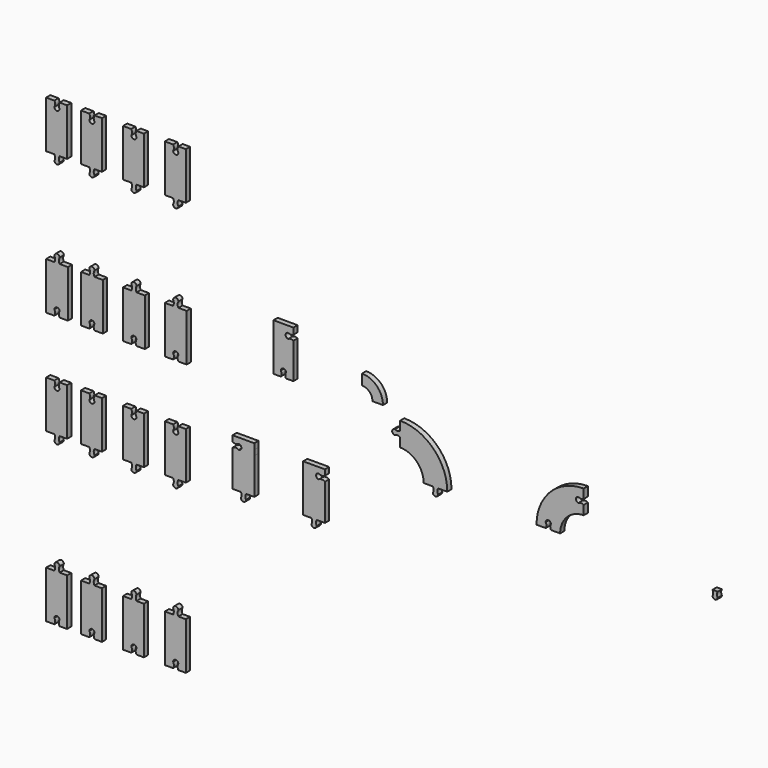
from build123d import *

# Parameters (mm, degrees)
F1_DEPTH = 25.4
F2_DEPTH = 25.4
F3_DEPTH = 25.4
F4_DEPTH = 25.4
F6_DEPTH = 25.4
F7_DEPTH = 25.4
F8_DEPTH = 25.4
F9_DEPTH = 25.4


# Not quite as in the source:
# - a feature names something its author has since deleted; it is built from what else it names


with BuildPart() as f1:
    # F0 (on Front) → F1 (new body)
    with BuildSketch(Plane.XZ):
        with BuildLine():
            Line((-45.9600600243, 819.565417695), (-82.0480443865, 819.565417695))
            ThreePointArc((-82.0480443865, 819.565417695), (-85.8930500594, 806.128817695), (-82.0480443865, 792.692217695))
            ThreePointArc((-82.0480443865, 792.692217695), (-94.7480443865, 779.992217695), (-107.4480443865, 792.692217695))
            ThreePointArc((-107.4480443865, 792.692217695), (-103.6030387136, 806.128817695), (-107.4480443865, 819.565417695))
            Line((-107.4480443865, 819.565417695), (-147.5600600243, 819.565417695))
            Line((-147.5600600243, 819.565417695), (-147.5600600243, 590.965417695))
            Line((-147.5600600243, 590.965417695), (-107.4480443865, 590.965417695))
            Line((-107.4480443865, 590.965417695), (-82.0480443865, 590.965417695))
            Line((-82.0480443865, 590.965417695), (-45.9600600243, 590.965417695))
            Line((-45.9600600243, 590.965417695), (-45.9600600243, 819.565417695))
        make_face()
    extrude(amount=F1_DEPTH)


with BuildPart() as f1b:
    # F0 (on Front) → F1, piece 2 (new body)
    with BuildSketch(Plane.XZ):
        with BuildLine():
            Line((21.4956142008, 590.965417695), (61.6076298386, 590.965417695))
            Line((61.6076298386, 590.965417695), (87.0076298386, 590.965417695))
            Line((87.0076298386, 590.965417695), (123.0956142008, 590.965417695))
            Line((123.0956142008, 590.965417695), (123.0956142008, 819.565417695))
            Line((123.0956142008, 819.565417695), (87.0076298386, 819.565417695))
            ThreePointArc((87.0076298386, 819.565417695), (83.1626241657, 806.128817695), (87.0076298386, 792.692217695))
            ThreePointArc((87.0076298386, 792.692217695), (74.3076298386, 779.992217695), (61.6076298386, 792.692217695))
            ThreePointArc((61.6076298386, 792.692217695), (65.4526355115, 806.128817695), (61.6076298386, 819.565417695))
            Line((61.6076298386, 819.565417695), (21.4956142008, 819.565417695))
            Line((21.4956142008, 819.565417695), (21.4956142008, 590.965417695))
        make_face()
    extrude(amount=F1_DEPTH)


with BuildPart() as f1c:
    # F0 (on Front) → F1, piece 3 (new body)
    with BuildSketch(Plane.XZ):
        with BuildLine():
            Line((264.7652149528, 590.965417695), (290.1652149528, 590.965417695))
            Line((290.1652149528, 590.965417695), (326.2531993151, 590.965417695))
            Line((326.2531993151, 590.965417695), (326.2531993151, 819.565417695))
            Line((326.2531993151, 819.565417695), (290.1652149528, 819.565417695))
            ThreePointArc((290.1652149528, 819.565417695), (286.3202092799, 806.128817695), (290.1652149528, 792.692217695))
            ThreePointArc((290.1652149528, 792.692217695), (277.4652149528, 779.992217695), (264.7652149528, 792.692217695))
            ThreePointArc((264.7652149528, 792.692217695), (268.6102206258, 806.128817695), (264.7652149528, 819.565417695))
            Line((264.7652149528, 819.565417695), (224.6531993151, 819.565417695))
            Line((224.6531993151, 819.565417695), (224.6531993151, 590.965417695))
            Line((224.6531993151, 590.965417695), (264.7652149528, 590.965417695))
        make_face()
    extrude(amount=F1_DEPTH)


with BuildPart() as f1d:
    # F0 (on Front) → F1, piece 4 (new body)
    with BuildSketch(Plane.XZ):
        with BuildLine():
            Line((427.3546077311, 590.965417695), (467.4666233689, 590.965417695))
            Line((467.4666233689, 590.965417695), (492.8666233689, 590.965417695))
            Line((492.8666233689, 590.965417695), (528.9546077311, 590.965417695))
            Line((528.9546077311, 590.965417695), (528.9546077311, 819.565417695))
            Line((528.9546077311, 819.565417695), (492.8666233689, 819.565417695))
            ThreePointArc((492.8666233689, 819.565417695), (489.0216176959, 806.128817695), (492.8666233689, 792.692217695))
            ThreePointArc((492.8666233689, 792.692217695), (480.1666233689, 779.992217695), (467.4666233689, 792.692217695))
            ThreePointArc((467.4666233689, 792.692217695), (471.3116290418, 806.128817695), (467.4666233689, 819.565417695))
            Line((467.4666233689, 819.565417695), (427.3546077311, 819.565417695))
            Line((427.3546077311, 819.565417695), (427.3546077311, 590.965417695))
        make_face()
    extrude(amount=F1_DEPTH)


with BuildPart() as f1e:
    # F0 (on Front) → F1, piece 5 (new body)
    with BuildSketch(Plane.XZ):
        with BuildLine():
            Line((492.8666233689, 131.5058790922), (467.4666233689, 131.5058790922))
            Line((467.4666233689, 131.5058790922), (427.3546077311, 131.5058790922))
            Line((427.3546077311, 131.5058790922), (427.3546077311, -97.0941209078))
            Line((427.3546077311, -97.0941209078), (467.4666233689, -97.0941209078))
            ThreePointArc((467.4666233689, -97.0941209078), (471.3116290418, -83.6575209078), (467.4666233689, -70.2209209078))
            ThreePointArc((467.4666233689, -70.2209209078), (480.1666233689, -57.5209209078), (492.8666233689, -70.2209209078))
            ThreePointArc((492.8666233689, -70.2209209078), (489.0216176959, -83.6575209078), (492.8666233689, -97.0941209078))
            Line((492.8666233689, -97.0941209078), (532.9786390066, -97.0941209078))
            Line((532.9786390066, -97.0941209078), (532.9786390066, 131.5058790922))
            Line((532.9786390066, 131.5058790922), (492.8666233689, 131.5058790922))
        make_face()
    extrude(amount=F1_DEPTH)


with BuildPart() as f1f:
    # F0 (on Front) → F1, piece 6 (new body)
    with BuildSketch(Plane.XZ):
        with BuildLine():
            ThreePointArc((264.7652149528, -70.2209209078), (277.4652149528, -57.5209209078), (290.1652149528, -70.2209209078))
            ThreePointArc((290.1652149528, -70.2209209078), (286.3202092799, -83.6575209078), (290.1652149528, -97.0941209078))
            Line((290.1652149528, -97.0941209078), (330.2772305906, -97.0941209078))
            Line((330.2772305906, -97.0941209078), (330.2772305906, 131.5058790922))
            Line((330.2772305906, 131.5058790922), (290.1652149528, 131.5058790922))
            Line((290.1652149528, 131.5058790922), (264.7652149528, 131.5058790922))
            Line((264.7652149528, 131.5058790922), (224.6531993151, 131.5058790922))
            Line((224.6531993151, 131.5058790922), (224.6531993151, -97.0941209078))
            Line((224.6531993151, -97.0941209078), (264.7652149528, -97.0941209078))
            ThreePointArc((264.7652149528, -97.0941209078), (268.6102206258, -83.6575209078), (264.7652149528, -70.2209209078))
        make_face()
    extrude(amount=F1_DEPTH)


with BuildPart() as f1g:
    # F0 (on Front) → F1, piece 7 (new body)
    with BuildSketch(Plane.XZ):
        with BuildLine():
            Line((21.4956142008, -97.0941209078), (61.6076298386, -97.0941209078))
            ThreePointArc((61.6076298386, -97.0941209078), (65.4526355115, -83.6575209078), (61.6076298386, -70.2209209078))
            ThreePointArc((61.6076298386, -70.2209209078), (74.3076298386, -57.5209209078), (87.0076298386, -70.2209209078))
            ThreePointArc((87.0076298386, -70.2209209078), (83.1626241657, -83.6575209078), (87.0076298386, -97.0941209078))
            Line((87.0076298386, -97.0941209078), (127.1196454763, -97.0941209078))
            Line((127.1196454763, -97.0941209078), (127.1196454763, 131.5058790922))
            Line((127.1196454763, 131.5058790922), (87.0076298386, 131.5058790922))
            Line((87.0076298386, 131.5058790922), (61.6076298386, 131.5058790922))
            Line((61.6076298386, 131.5058790922), (21.4956142008, 131.5058790922))
            Line((21.4956142008, 131.5058790922), (21.4956142008, -97.0941209078))
        make_face()
    extrude(amount=F1_DEPTH)


with BuildPart() as f1h:
    # F0 (on Front) → F1, piece 8 (new body)
    with BuildSketch(Plane.XZ):
        with BuildLine():
            Line((-107.4480443865, 131.5058790922), (-147.5600600243, 131.5058790922))
            Line((-147.5600600243, 131.5058790922), (-147.5600600243, -97.0941209078))
            Line((-147.5600600243, -97.0941209078), (-107.4480443865, -97.0941209078))
            ThreePointArc((-107.4480443865, -97.0941209078), (-103.6030387136, -83.6575209078), (-107.4480443865, -70.2209209078))
            ThreePointArc((-107.4480443865, -70.2209209078), (-94.7480443865, -57.5209209078), (-82.0480443865, -70.2209209078))
            ThreePointArc((-82.0480443865, -70.2209209078), (-85.8930500594, -83.6575209078), (-82.0480443865, -97.0941209078))
            Line((-82.0480443865, -97.0941209078), (-41.9360287488, -97.0941209078))
            Line((-41.9360287488, -97.0941209078), (-41.9360287488, 131.5058790922))
            Line((-41.9360287488, 131.5058790922), (-82.0480443865, 131.5058790922))
            Line((-82.0480443865, 131.5058790922), (-107.4480443865, 131.5058790922))
        make_face()
    extrude(amount=F1_DEPTH)


with BuildPart() as f1i:
    # F0 (on Front) → F1, piece 9 (new body)
    with BuildSketch(Plane.XZ):
        with BuildLine():
            ThreePointArc((-107.4480443865, -400.1181687243), (-103.6030387136, -386.6815687243), (-107.4480443865, -373.2449687243))
            Line((-107.4480443865, -373.2449687243), (-147.5600600243, -373.2449687243))
            Line((-147.5600600243, -373.2449687243), (-147.5600600243, -601.8449687243))
            Line((-147.5600600243, -601.8449687243), (-107.4480443865, -601.8449687243))
            Line((-107.4480443865, -601.8449687243), (-82.0480443865, -601.8449687243))
            Line((-82.0480443865, -601.8449687243), (-45.9600600243, -601.8449687243))
            Line((-45.9600600243, -601.8449687243), (-45.9600600243, -373.2449687243))
            Line((-45.9600600243, -373.2449687243), (-82.0480443865, -373.2449687243))
            ThreePointArc((-82.0480443865, -373.2449687243), (-85.8930500594, -386.6815687243), (-82.0480443865, -400.1181687243))
            ThreePointArc((-82.0480443865, -400.1181687243), (-94.7480443865, -412.8181687243), (-107.4480443865, -400.1181687243))
        make_face()
    extrude(amount=F1_DEPTH)


with BuildPart() as f1j:
    # F0 (on Front) → F1, piece 10 (new body)
    with BuildSketch(Plane.XZ):
        with BuildLine():
            ThreePointArc((61.6076298386, -400.1181687243), (65.4526355115, -386.6815687243), (61.6076298386, -373.2449687243))
            Line((61.6076298386, -373.2449687243), (21.4956142008, -373.2449687243))
            Line((21.4956142008, -373.2449687243), (21.4956142008, -601.8449687243))
            Line((21.4956142008, -601.8449687243), (61.6076298386, -601.8449687243))
            Line((61.6076298386, -601.8449687243), (87.0076298386, -601.8449687243))
            Line((87.0076298386, -601.8449687243), (123.0956142008, -601.8449687243))
            Line((123.0956142008, -601.8449687243), (123.0956142008, -373.2449687243))
            Line((123.0956142008, -373.2449687243), (87.0076298386, -373.2449687243))
            ThreePointArc((87.0076298386, -373.2449687243), (83.1626241657, -386.6815687243), (87.0076298386, -400.1181687243))
            ThreePointArc((87.0076298386, -400.1181687243), (74.3076298386, -412.8181687243), (61.6076298386, -400.1181687243))
        make_face()
    extrude(amount=F1_DEPTH)


with BuildPart() as f1k:
    # F0 (on Front) → F1, piece 11 (new body)
    with BuildSketch(Plane.XZ):
        with BuildLine():
            ThreePointArc((264.7652149528, -400.1181687243), (268.6102206258, -386.6815687243), (264.7652149528, -373.2449687243))
            Line((264.7652149528, -373.2449687243), (224.6531993151, -373.2449687243))
            Line((224.6531993151, -373.2449687243), (224.6531993151, -601.8449687243))
            Line((224.6531993151, -601.8449687243), (264.7652149528, -601.8449687243))
            Line((264.7652149528, -601.8449687243), (290.1652149528, -601.8449687243))
            Line((290.1652149528, -601.8449687243), (326.2531993151, -601.8449687243))
            Line((326.2531993151, -601.8449687243), (326.2531993151, -373.2449687243))
            Line((326.2531993151, -373.2449687243), (290.1652149528, -373.2449687243))
            ThreePointArc((290.1652149528, -373.2449687243), (286.3202092799, -386.6815687243), (290.1652149528, -400.1181687243))
            ThreePointArc((290.1652149528, -400.1181687243), (277.4652149528, -412.8181687243), (264.7652149528, -400.1181687243))
        make_face()
    extrude(amount=F1_DEPTH)


with BuildPart() as f1l:
    # F0 (on Front) → F1, piece 12 (new body)
    with BuildSketch(Plane.XZ):
        with BuildLine():
            Line((528.9546077311, -373.2449687243), (492.8666233689, -373.2449687243))
            ThreePointArc((492.8666233689, -373.2449687243), (489.0216176959, -386.6815687243), (492.8666233689, -400.1181687243))
            ThreePointArc((492.8666233689, -400.1181687243), (480.1666233689, -412.8181687243), (467.4666233689, -400.1181687243))
            ThreePointArc((467.4666233689, -400.1181687243), (471.3116290418, -386.6815687243), (467.4666233689, -373.2449687243))
            Line((467.4666233689, -373.2449687243), (427.3546077311, -373.2449687243))
            Line((427.3546077311, -373.2449687243), (427.3546077311, -601.8449687243))
            Line((427.3546077311, -601.8449687243), (467.4666233689, -601.8449687243))
            Line((467.4666233689, -601.8449687243), (492.8666233689, -601.8449687243))
            Line((492.8666233689, -601.8449687243), (528.9546077311, -601.8449687243))
            Line((528.9546077311, -601.8449687243), (528.9546077311, -373.2449687243))
        make_face()
    extrude(amount=F1_DEPTH)


with BuildPart() as f1m:
    # F0 (on Front) → F1, piece 13 (new body)
    with BuildSketch(Plane.XZ):
        with BuildLine():
            ThreePointArc((492.8666233689, -1385.466757881), (489.0216176959, -1398.903357881), (492.8666233689, -1412.339957881))
            Line((492.8666233689, -1412.339957881), (528.9546077311, -1412.339957881))
            Line((528.9546077311, -1412.339957881), (528.9546077311, -1183.739957881))
            Line((528.9546077311, -1183.739957881), (492.8666233689, -1183.739957881))
            Line((492.8666233689, -1183.739957881), (467.4666233689, -1183.739957881))
            Line((467.4666233689, -1183.739957881), (427.3546077311, -1183.739957881))
            Line((427.3546077311, -1183.739957881), (427.3546077311, -1412.339957881))
            Line((427.3546077311, -1412.339957881), (467.4666233689, -1412.339957881))
            ThreePointArc((467.4666233689, -1412.339957881), (471.3116290418, -1398.903357881), (467.4666233689, -1385.466757881))
            ThreePointArc((467.4666233689, -1385.466757881), (480.1666233689, -1372.766757881), (492.8666233689, -1385.466757881))
        make_face()
    extrude(amount=F1_DEPTH)


with BuildPart() as f1n:
    # F0 (on Front) → F1, piece 14 (new body)
    with BuildSketch(Plane.XZ):
        with BuildLine():
            ThreePointArc((264.7652149528, -1385.466757881), (277.4652149528, -1372.766757881), (290.1652149528, -1385.466757881))
            ThreePointArc((290.1652149528, -1385.466757881), (286.3202092799, -1398.903357881), (290.1652149528, -1412.339957881))
            Line((290.1652149528, -1412.339957881), (326.2531993151, -1412.339957881))
            Line((326.2531993151, -1412.339957881), (326.2531993151, -1183.739957881))
            Line((326.2531993151, -1183.739957881), (290.1652149528, -1183.739957881))
            Line((290.1652149528, -1183.739957881), (264.7652149528, -1183.739957881))
            Line((264.7652149528, -1183.739957881), (224.6531993151, -1183.739957881))
            Line((224.6531993151, -1183.739957881), (224.6531993151, -1412.339957881))
            Line((224.6531993151, -1412.339957881), (264.7652149528, -1412.339957881))
            ThreePointArc((264.7652149528, -1412.339957881), (268.6102206258, -1398.903357881), (264.7652149528, -1385.466757881))
        make_face()
    extrude(amount=F1_DEPTH)


with BuildPart() as f1o:
    # F0 (on Front) → F1, piece 15 (new body)
    with BuildSketch(Plane.XZ):
        with BuildLine():
            Line((87.0076298386, -1183.739957881), (61.6076298386, -1183.739957881))
            Line((61.6076298386, -1183.739957881), (21.4956142008, -1183.739957881))
            Line((21.4956142008, -1183.739957881), (21.4956142008, -1412.339957881))
            Line((21.4956142008, -1412.339957881), (61.6076298386, -1412.339957881))
            ThreePointArc((61.6076298386, -1412.339957881), (65.4526355115, -1398.903357881), (61.6076298386, -1385.466757881))
            ThreePointArc((61.6076298386, -1385.466757881), (74.3076298386, -1372.766757881), (87.0076298386, -1385.466757881))
            ThreePointArc((87.0076298386, -1385.466757881), (83.1626241657, -1398.903357881), (87.0076298386, -1412.339957881))
            Line((87.0076298386, -1412.339957881), (123.0956142008, -1412.339957881))
            Line((123.0956142008, -1412.339957881), (123.0956142008, -1183.739957881))
            Line((123.0956142008, -1183.739957881), (87.0076298386, -1183.739957881))
        make_face()
    extrude(amount=F1_DEPTH)


with BuildPart() as f1p:
    # F0 (on Front) → F1, piece 16 (new body)
    with BuildSketch(Plane.XZ):
        with BuildLine():
            ThreePointArc((-107.4480443865, -1385.466757881), (-94.7480443865, -1372.766757881), (-82.0480443865, -1385.466757881))
            ThreePointArc((-82.0480443865, -1385.466757881), (-85.8930500594, -1398.903357881), (-82.0480443865, -1412.339957881))
            Line((-82.0480443865, -1412.339957881), (-45.9600600243, -1412.339957881))
            Line((-45.9600600243, -1412.339957881), (-45.9600600243, -1183.739957881))
            Line((-45.9600600243, -1183.739957881), (-82.0480443865, -1183.739957881))
            Line((-82.0480443865, -1183.739957881), (-107.4480443865, -1183.739957881))
            Line((-107.4480443865, -1183.739957881), (-147.5600600243, -1183.739957881))
            Line((-147.5600600243, -1183.739957881), (-147.5600600243, -1412.339957881))
            Line((-147.5600600243, -1412.339957881), (-107.4480443865, -1412.339957881))
            ThreePointArc((-107.4480443865, -1412.339957881), (-103.6030387136, -1398.903357881), (-107.4480443865, -1385.466757881))
        make_face()
    extrude(amount=F1_DEPTH)


with BuildPart() as f2:
    # F0 (on Front) → F2 (new body)
    with BuildSketch(Plane.XZ):
        with BuildLine():
            ThreePointArc((492.8666233689, 158.3865135908), (480.1666233689, 171.0865135908), (467.4666233689, 158.3865135908))
            ThreePointArc((467.4666233689, 158.3865135908), (470.8542959546, 144.9461963415), (467.4666233689, 131.5058790922))
            Line((467.4666233689, 131.5058790922), (492.8666233689, 131.5058790922))
            ThreePointArc((492.8666233689, 131.5058790922), (489.0193000527, 144.9461963415), (492.8666233689, 158.3865135908))
        make_face()
    extrude(amount=F2_DEPTH)


with BuildPart() as f2b:
    # F0 (on Front) → F2, piece 2 (new body)
    with BuildSketch(Plane.XZ):
        with BuildLine():
            Line((264.7652149528, 131.5058790922), (290.1652149528, 131.5058790922))
            ThreePointArc((290.1652149528, 131.5058790922), (286.7775423671, 144.9461963415), (290.1652149528, 158.3865135908))
            ThreePointArc((290.1652149528, 158.3865135908), (277.4652149528, 171.0865135908), (264.7652149528, 158.3865135908))
            ThreePointArc((264.7652149528, 158.3865135908), (268.612538269, 144.9461963415), (264.7652149528, 131.5058790922))
        make_face()
    extrude(amount=F2_DEPTH)


with BuildPart() as f2c:
    # F0 (on Front) → F2, piece 3 (new body)
    with BuildSketch(Plane.XZ):
        with BuildLine():
            ThreePointArc((61.6076298386, 158.3865135908), (64.9953024243, 144.9461963415), (61.6076298386, 131.5058790922))
            Line((61.6076298386, 131.5058790922), (87.0076298386, 131.5058790922))
            ThreePointArc((87.0076298386, 131.5058790922), (83.1603065224, 144.9461963415), (87.0076298386, 158.3865135908))
            ThreePointArc((87.0076298386, 158.3865135908), (74.3076298386, 171.0865135908), (61.6076298386, 158.3865135908))
        make_face()
    extrude(amount=F2_DEPTH)


with BuildPart() as f2d:
    # F0 (on Front) → F2, piece 4 (new body)
    with BuildSketch(Plane.XZ):
        with BuildLine():
            ThreePointArc((-107.4480443865, 158.3865135908), (-103.6007210703, 144.9461963415), (-107.4480443865, 131.5058790922))
            Line((-107.4480443865, 131.5058790922), (-82.0480443865, 131.5058790922))
            ThreePointArc((-82.0480443865, 131.5058790922), (-85.4357169722, 144.9461963415), (-82.0480443865, 158.3865135908))
            ThreePointArc((-82.0480443865, 158.3865135908), (-94.7480443865, 171.0865135908), (-107.4480443865, 158.3865135908))
        make_face()
    extrude(amount=F2_DEPTH)


with BuildPart() as f2e:
    # F0 (on Front) → F2, piece 5 (new body)
    with BuildSketch(Plane.XZ):
        with BuildLine():
            Line((-82.0480443865, -601.8449687243), (-107.4480443865, -601.8449687243))
            ThreePointArc((-107.4480443865, -601.8449687243), (-103.6007210703, -615.2852859735), (-107.4480443865, -628.7256032228))
            ThreePointArc((-107.4480443865, -628.7256032228), (-94.7480443865, -641.4256032228), (-82.0480443865, -628.7256032228))
            ThreePointArc((-82.0480443865, -628.7256032228), (-85.4357169722, -615.2852859735), (-82.0480443865, -601.8449687243))
        make_face()
    extrude(amount=F2_DEPTH)


with BuildPart() as f2f:
    # F0 (on Front) → F2, piece 6 (new body)
    with BuildSketch(Plane.XZ):
        with BuildLine():
            Line((87.0076298386, -601.8449687243), (61.6076298386, -601.8449687243))
            ThreePointArc((61.6076298386, -601.8449687243), (64.9953024243, -615.2852859735), (61.6076298386, -628.7256032228))
            ThreePointArc((61.6076298386, -628.7256032228), (74.3076298386, -641.4256032228), (87.0076298386, -628.7256032228))
            ThreePointArc((87.0076298386, -628.7256032228), (83.1603065224, -615.2852859735), (87.0076298386, -601.8449687243))
        make_face()
    extrude(amount=F2_DEPTH)


with BuildPart() as f2g:
    # F0 (on Front) → F2, piece 7 (new body)
    with BuildSketch(Plane.XZ):
        with BuildLine():
            Line((290.1652149528, -601.8449687243), (264.7652149528, -601.8449687243))
            ThreePointArc((264.7652149528, -601.8449687243), (268.612538269, -615.2852859735), (264.7652149528, -628.7256032228))
            ThreePointArc((264.7652149528, -628.7256032228), (277.4652149528, -641.4256032228), (290.1652149528, -628.7256032228))
            ThreePointArc((290.1652149528, -628.7256032228), (286.7775423671, -615.2852859735), (290.1652149528, -601.8449687243))
        make_face()
    extrude(amount=F2_DEPTH)


with BuildPart() as f2h:
    # F0 (on Front) → F2, piece 8 (new body)
    with BuildSketch(Plane.XZ):
        with BuildLine():
            ThreePointArc((492.8666233689, -628.7256032228), (489.0193000527, -615.2852859735), (492.8666233689, -601.8449687243))
            Line((492.8666233689, -601.8449687243), (467.4666233689, -601.8449687243))
            ThreePointArc((467.4666233689, -601.8449687243), (470.8542959546, -615.2852859735), (467.4666233689, -628.7256032228))
            ThreePointArc((467.4666233689, -628.7256032228), (480.1666233689, -641.4256032228), (492.8666233689, -628.7256032228))
        make_face()
    extrude(amount=F2_DEPTH)


with BuildPart() as f2i:
    # F0 (on Front) → F2, piece 9 (new body)
    with BuildSketch(Plane.XZ):
        with BuildLine():
            Line((467.4666233689, -1183.739957881), (492.8666233689, -1183.739957881))
            ThreePointArc((492.8666233689, -1183.739957881), (489.0193000527, -1170.2996406317), (492.8666233689, -1156.8593233824))
            ThreePointArc((492.8666233689, -1156.8593233824), (480.1666233689, -1144.1593233824), (467.4666233689, -1156.8593233824))
            ThreePointArc((467.4666233689, -1156.8593233824), (470.8542959546, -1170.2996406317), (467.4666233689, -1183.739957881))
        make_face()
    extrude(amount=F2_DEPTH)


with BuildPart() as f2j:
    # F0 (on Front) → F2, piece 10 (new body)
    with BuildSketch(Plane.XZ):
        with BuildLine():
            Line((264.7652149528, -1183.739957881), (290.1652149528, -1183.739957881))
            ThreePointArc((290.1652149528, -1183.739957881), (286.7775423671, -1170.2996406317), (290.1652149528, -1156.8593233824))
            ThreePointArc((290.1652149528, -1156.8593233824), (277.4652149528, -1144.1593233824), (264.7652149528, -1156.8593233824))
            ThreePointArc((264.7652149528, -1156.8593233824), (268.612538269, -1170.2996406317), (264.7652149528, -1183.739957881))
        make_face()
    extrude(amount=F2_DEPTH)


with BuildPart() as f2k:
    # F0 (on Front) → F2, piece 11 (new body)
    with BuildSketch(Plane.XZ):
        with BuildLine():
            ThreePointArc((87.0076298386, -1156.8593233824), (74.3076298386, -1144.1593233824), (61.6076298386, -1156.8593233824))
            ThreePointArc((61.6076298386, -1156.8593233824), (64.9953024243, -1170.2996406317), (61.6076298386, -1183.739957881))
            Line((61.6076298386, -1183.739957881), (87.0076298386, -1183.739957881))
            ThreePointArc((87.0076298386, -1183.739957881), (83.1603065224, -1170.2996406317), (87.0076298386, -1156.8593233824))
        make_face()
    extrude(amount=F2_DEPTH)


with BuildPart() as f2l:
    # F0 (on Front) → F2, piece 12 (new body)
    with BuildSketch(Plane.XZ):
        with BuildLine():
            Line((-107.4480443865, -1183.739957881), (-82.0480443865, -1183.739957881))
            ThreePointArc((-82.0480443865, -1183.739957881), (-85.4357169722, -1170.2996406317), (-82.0480443865, -1156.8593233824))
            ThreePointArc((-82.0480443865, -1156.8593233824), (-94.7480443865, -1144.1593233824), (-107.4480443865, -1156.8593233824))
            ThreePointArc((-107.4480443865, -1156.8593233824), (-103.6007210703, -1170.2996406317), (-107.4480443865, -1183.739957881))
        make_face()
    extrude(amount=F2_DEPTH)


with BuildPart() as f2m:
    # F0 (on Front) → F2, piece 13 (new body)
    with BuildSketch(Plane.XZ):
        with BuildLine():
            ThreePointArc((467.4666233689, 590.965417695), (470.8542959546, 577.5251004457), (467.4666233689, 564.0847831964))
            ThreePointArc((467.4666233689, 564.0847831964), (480.1666233689, 551.3847831964), (492.8666233689, 564.0847831964))
            ThreePointArc((492.8666233689, 564.0847831964), (489.0193000527, 577.5251004457), (492.8666233689, 590.965417695))
            Line((492.8666233689, 590.965417695), (467.4666233689, 590.965417695))
        make_face()
    extrude(amount=F2_DEPTH)


with BuildPart() as f2n:
    # F0 (on Front) → F2, piece 14 (new body)
    with BuildSketch(Plane.XZ):
        with BuildLine():
            ThreePointArc((264.7652149528, 564.0847831964), (277.4652149528, 551.3847831964), (290.1652149528, 564.0847831964))
            ThreePointArc((290.1652149528, 564.0847831964), (286.7775423671, 577.5251004457), (290.1652149528, 590.965417695))
            Line((290.1652149528, 590.965417695), (264.7652149528, 590.965417695))
            ThreePointArc((264.7652149528, 590.965417695), (268.612538269, 577.5251004457), (264.7652149528, 564.0847831964))
        make_face()
    extrude(amount=F2_DEPTH)


with BuildPart() as f2o:
    # F0 (on Front) → F2, piece 15 (new body)
    with BuildSketch(Plane.XZ):
        with BuildLine():
            ThreePointArc((61.6076298386, 590.965417695), (64.9953024243, 577.5251004457), (61.6076298386, 564.0847831964))
            ThreePointArc((61.6076298386, 564.0847831964), (74.3076298386, 551.3847831964), (87.0076298386, 564.0847831964))
            ThreePointArc((87.0076298386, 564.0847831964), (83.1603065224, 577.5251004457), (87.0076298386, 590.965417695))
            Line((87.0076298386, 590.965417695), (61.6076298386, 590.965417695))
        make_face()
    extrude(amount=F2_DEPTH)


with BuildPart() as f2p:
    # F0 (on Front) → F2, piece 16 (new body)
    with BuildSketch(Plane.XZ):
        with BuildLine():
            ThreePointArc((-82.0480443865, 564.0847831964), (-85.4357169722, 577.5251004457), (-82.0480443865, 590.965417695))
            Line((-82.0480443865, 590.965417695), (-107.4480443865, 590.965417695))
            ThreePointArc((-107.4480443865, 590.965417695), (-103.6007210703, 577.5251004457), (-107.4480443865, 564.0847831964))
            ThreePointArc((-107.4480443865, 564.0847831964), (-94.7480443865, 551.3847831964), (-82.0480443865, 564.0847831964))
        make_face()
    extrude(amount=F2_DEPTH)


with BuildPart() as f3:
    # F0 (on Front) → F3 (new body)
    with BuildSketch(Plane.XZ):
        with BuildLine():
            Line((-107.4480443865, 131.5058790922), (-147.5600600243, 131.5058790922))
            Line((-147.5600600243, 131.5058790922), (-147.5600600243, -97.0941209078))
            Line((-147.5600600243, -97.0941209078), (-107.4480443865, -97.0941209078))
            ThreePointArc((-107.4480443865, -97.0941209078), (-103.6030387136, -83.6575209078), (-107.4480443865, -70.2209209078))
            ThreePointArc((-107.4480443865, -70.2209209078), (-94.7480443865, -57.5209209078), (-82.0480443865, -70.2209209078))
            ThreePointArc((-82.0480443865, -70.2209209078), (-85.8930500594, -83.6575209078), (-82.0480443865, -97.0941209078))
            Line((-82.0480443865, -97.0941209078), (-41.9360287488, -97.0941209078))
            Line((-41.9360287488, -97.0941209078), (-41.9360287488, 131.5058790922))
            Line((-41.9360287488, 131.5058790922), (-82.0480443865, 131.5058790922))
            Line((-82.0480443865, 131.5058790922), (-107.4480443865, 131.5058790922))
        make_face()
        with BuildLine():
            ThreePointArc((-107.4480443865, 158.3865135908), (-103.6007210703, 144.9461963415), (-107.4480443865, 131.5058790922))
            Line((-107.4480443865, 131.5058790922), (-82.0480443865, 131.5058790922))
            ThreePointArc((-82.0480443865, 131.5058790922), (-85.4357169722, 144.9461963415), (-82.0480443865, 158.3865135908))
            ThreePointArc((-82.0480443865, 158.3865135908), (-94.7480443865, 171.0865135908), (-107.4480443865, 158.3865135908))
        make_face()
    extrude(amount=F3_DEPTH)


with BuildPart() as f3b:
    # F0 (on Front) → F3, piece 2 (new body)
    with BuildSketch(Plane.XZ):
        with BuildLine():
            Line((21.4956142008, -97.0941209078), (61.6076298386, -97.0941209078))
            ThreePointArc((61.6076298386, -97.0941209078), (65.4526355115, -83.6575209078), (61.6076298386, -70.2209209078))
            ThreePointArc((61.6076298386, -70.2209209078), (74.3076298386, -57.5209209078), (87.0076298386, -70.2209209078))
            ThreePointArc((87.0076298386, -70.2209209078), (83.1626241657, -83.6575209078), (87.0076298386, -97.0941209078))
            Line((87.0076298386, -97.0941209078), (127.1196454763, -97.0941209078))
            Line((127.1196454763, -97.0941209078), (127.1196454763, 131.5058790922))
            Line((127.1196454763, 131.5058790922), (87.0076298386, 131.5058790922))
            Line((87.0076298386, 131.5058790922), (61.6076298386, 131.5058790922))
            Line((61.6076298386, 131.5058790922), (21.4956142008, 131.5058790922))
            Line((21.4956142008, 131.5058790922), (21.4956142008, -97.0941209078))
        make_face()
        with BuildLine():
            ThreePointArc((61.6076298386, 158.3865135908), (64.9953024243, 144.9461963415), (61.6076298386, 131.5058790922))
            Line((61.6076298386, 131.5058790922), (87.0076298386, 131.5058790922))
            ThreePointArc((87.0076298386, 131.5058790922), (83.1603065224, 144.9461963415), (87.0076298386, 158.3865135908))
            ThreePointArc((87.0076298386, 158.3865135908), (74.3076298386, 171.0865135908), (61.6076298386, 158.3865135908))
        make_face()
    extrude(amount=F3_DEPTH)


with BuildPart() as f3c:
    # F0 (on Front) → F3, piece 3 (new body)
    with BuildSketch(Plane.XZ):
        with BuildLine():
            ThreePointArc((264.7652149528, -70.2209209078), (277.4652149528, -57.5209209078), (290.1652149528, -70.2209209078))
            ThreePointArc((290.1652149528, -70.2209209078), (286.3202092799, -83.6575209078), (290.1652149528, -97.0941209078))
            Line((290.1652149528, -97.0941209078), (330.2772305906, -97.0941209078))
            Line((330.2772305906, -97.0941209078), (330.2772305906, 131.5058790922))
            Line((330.2772305906, 131.5058790922), (290.1652149528, 131.5058790922))
            Line((290.1652149528, 131.5058790922), (264.7652149528, 131.5058790922))
            Line((264.7652149528, 131.5058790922), (224.6531993151, 131.5058790922))
            Line((224.6531993151, 131.5058790922), (224.6531993151, -97.0941209078))
            Line((224.6531993151, -97.0941209078), (264.7652149528, -97.0941209078))
            ThreePointArc((264.7652149528, -97.0941209078), (268.6102206258, -83.6575209078), (264.7652149528, -70.2209209078))
        make_face()
        with BuildLine():
            Line((264.7652149528, 131.5058790922), (290.1652149528, 131.5058790922))
            ThreePointArc((290.1652149528, 131.5058790922), (286.7775423671, 144.9461963415), (290.1652149528, 158.3865135908))
            ThreePointArc((290.1652149528, 158.3865135908), (277.4652149528, 171.0865135908), (264.7652149528, 158.3865135908))
            ThreePointArc((264.7652149528, 158.3865135908), (268.612538269, 144.9461963415), (264.7652149528, 131.5058790922))
        make_face()
    extrude(amount=F3_DEPTH)


with BuildPart() as f3d:
    # F0 (on Front) → F3, piece 4 (new body)
    with BuildSketch(Plane.XZ):
        with BuildLine():
            ThreePointArc((492.8666233689, 158.3865135908), (480.1666233689, 171.0865135908), (467.4666233689, 158.3865135908))
            ThreePointArc((467.4666233689, 158.3865135908), (470.8542959546, 144.9461963415), (467.4666233689, 131.5058790922))
            Line((467.4666233689, 131.5058790922), (492.8666233689, 131.5058790922))
            ThreePointArc((492.8666233689, 131.5058790922), (489.0193000527, 144.9461963415), (492.8666233689, 158.3865135908))
        make_face()
        with BuildLine():
            Line((492.8666233689, 131.5058790922), (467.4666233689, 131.5058790922))
            Line((467.4666233689, 131.5058790922), (427.3546077311, 131.5058790922))
            Line((427.3546077311, 131.5058790922), (427.3546077311, -97.0941209078))
            Line((427.3546077311, -97.0941209078), (467.4666233689, -97.0941209078))
            ThreePointArc((467.4666233689, -97.0941209078), (471.3116290418, -83.6575209078), (467.4666233689, -70.2209209078))
            ThreePointArc((467.4666233689, -70.2209209078), (480.1666233689, -57.5209209078), (492.8666233689, -70.2209209078))
            ThreePointArc((492.8666233689, -70.2209209078), (489.0216176959, -83.6575209078), (492.8666233689, -97.0941209078))
            Line((492.8666233689, -97.0941209078), (532.9786390066, -97.0941209078))
            Line((532.9786390066, -97.0941209078), (532.9786390066, 131.5058790922))
            Line((532.9786390066, 131.5058790922), (492.8666233689, 131.5058790922))
        make_face()
    extrude(amount=F3_DEPTH)


with BuildPart() as f3e:
    # F0 (on Front) → F3, piece 5 (new body)
    with BuildSketch(Plane.XZ):
        with BuildLine():
            ThreePointArc((-107.4480443865, -400.1181687243), (-103.6030387136, -386.6815687243), (-107.4480443865, -373.2449687243))
            Line((-107.4480443865, -373.2449687243), (-147.5600600243, -373.2449687243))
            Line((-147.5600600243, -373.2449687243), (-147.5600600243, -601.8449687243))
            Line((-147.5600600243, -601.8449687243), (-107.4480443865, -601.8449687243))
            Line((-107.4480443865, -601.8449687243), (-82.0480443865, -601.8449687243))
            Line((-82.0480443865, -601.8449687243), (-45.9600600243, -601.8449687243))
            Line((-45.9600600243, -601.8449687243), (-45.9600600243, -373.2449687243))
            Line((-45.9600600243, -373.2449687243), (-82.0480443865, -373.2449687243))
            ThreePointArc((-82.0480443865, -373.2449687243), (-85.8930500594, -386.6815687243), (-82.0480443865, -400.1181687243))
            ThreePointArc((-82.0480443865, -400.1181687243), (-94.7480443865, -412.8181687243), (-107.4480443865, -400.1181687243))
        make_face()
        with BuildLine():
            Line((-82.0480443865, -601.8449687243), (-107.4480443865, -601.8449687243))
            ThreePointArc((-107.4480443865, -601.8449687243), (-103.6007210703, -615.2852859735), (-107.4480443865, -628.7256032228))
            ThreePointArc((-107.4480443865, -628.7256032228), (-94.7480443865, -641.4256032228), (-82.0480443865, -628.7256032228))
            ThreePointArc((-82.0480443865, -628.7256032228), (-85.4357169722, -615.2852859735), (-82.0480443865, -601.8449687243))
        make_face()
    extrude(amount=F3_DEPTH)


with BuildPart() as f3f:
    # F0 (on Front) → F3, piece 6 (new body)
    with BuildSketch(Plane.XZ):
        with BuildLine():
            ThreePointArc((264.7652149528, -400.1181687243), (268.6102206258, -386.6815687243), (264.7652149528, -373.2449687243))
            Line((264.7652149528, -373.2449687243), (224.6531993151, -373.2449687243))
            Line((224.6531993151, -373.2449687243), (224.6531993151, -601.8449687243))
            Line((224.6531993151, -601.8449687243), (264.7652149528, -601.8449687243))
            Line((264.7652149528, -601.8449687243), (290.1652149528, -601.8449687243))
            Line((290.1652149528, -601.8449687243), (326.2531993151, -601.8449687243))
            Line((326.2531993151, -601.8449687243), (326.2531993151, -373.2449687243))
            Line((326.2531993151, -373.2449687243), (290.1652149528, -373.2449687243))
            ThreePointArc((290.1652149528, -373.2449687243), (286.3202092799, -386.6815687243), (290.1652149528, -400.1181687243))
            ThreePointArc((290.1652149528, -400.1181687243), (277.4652149528, -412.8181687243), (264.7652149528, -400.1181687243))
        make_face()
        with BuildLine():
            Line((290.1652149528, -601.8449687243), (264.7652149528, -601.8449687243))
            ThreePointArc((264.7652149528, -601.8449687243), (268.612538269, -615.2852859735), (264.7652149528, -628.7256032228))
            ThreePointArc((264.7652149528, -628.7256032228), (277.4652149528, -641.4256032228), (290.1652149528, -628.7256032228))
            ThreePointArc((290.1652149528, -628.7256032228), (286.7775423671, -615.2852859735), (290.1652149528, -601.8449687243))
        make_face()
    extrude(amount=F3_DEPTH)


with BuildPart() as f3g:
    # F0 (on Front) → F3, piece 7 (new body)
    with BuildSketch(Plane.XZ):
        with BuildLine():
            ThreePointArc((61.6076298386, -400.1181687243), (65.4526355115, -386.6815687243), (61.6076298386, -373.2449687243))
            Line((61.6076298386, -373.2449687243), (21.4956142008, -373.2449687243))
            Line((21.4956142008, -373.2449687243), (21.4956142008, -601.8449687243))
            Line((21.4956142008, -601.8449687243), (61.6076298386, -601.8449687243))
            Line((61.6076298386, -601.8449687243), (87.0076298386, -601.8449687243))
            Line((87.0076298386, -601.8449687243), (123.0956142008, -601.8449687243))
            Line((123.0956142008, -601.8449687243), (123.0956142008, -373.2449687243))
            Line((123.0956142008, -373.2449687243), (87.0076298386, -373.2449687243))
            ThreePointArc((87.0076298386, -373.2449687243), (83.1626241657, -386.6815687243), (87.0076298386, -400.1181687243))
            ThreePointArc((87.0076298386, -400.1181687243), (74.3076298386, -412.8181687243), (61.6076298386, -400.1181687243))
        make_face()
        with BuildLine():
            Line((87.0076298386, -601.8449687243), (61.6076298386, -601.8449687243))
            ThreePointArc((61.6076298386, -601.8449687243), (64.9953024243, -615.2852859735), (61.6076298386, -628.7256032228))
            ThreePointArc((61.6076298386, -628.7256032228), (74.3076298386, -641.4256032228), (87.0076298386, -628.7256032228))
            ThreePointArc((87.0076298386, -628.7256032228), (83.1603065224, -615.2852859735), (87.0076298386, -601.8449687243))
        make_face()
    extrude(amount=F3_DEPTH)


with BuildPart() as f3h:
    # F0 (on Front) → F3, piece 8 (new body)
    with BuildSketch(Plane.XZ):
        with BuildLine():
            Line((528.9546077311, -373.2449687243), (492.8666233689, -373.2449687243))
            ThreePointArc((492.8666233689, -373.2449687243), (489.0216176959, -386.6815687243), (492.8666233689, -400.1181687243))
            ThreePointArc((492.8666233689, -400.1181687243), (480.1666233689, -412.8181687243), (467.4666233689, -400.1181687243))
            ThreePointArc((467.4666233689, -400.1181687243), (471.3116290418, -386.6815687243), (467.4666233689, -373.2449687243))
            Line((467.4666233689, -373.2449687243), (427.3546077311, -373.2449687243))
            Line((427.3546077311, -373.2449687243), (427.3546077311, -601.8449687243))
            Line((427.3546077311, -601.8449687243), (467.4666233689, -601.8449687243))
            Line((467.4666233689, -601.8449687243), (492.8666233689, -601.8449687243))
            Line((492.8666233689, -601.8449687243), (528.9546077311, -601.8449687243))
            Line((528.9546077311, -601.8449687243), (528.9546077311, -373.2449687243))
        make_face()
        with BuildLine():
            ThreePointArc((492.8666233689, -628.7256032228), (489.0193000527, -615.2852859735), (492.8666233689, -601.8449687243))
            Line((492.8666233689, -601.8449687243), (467.4666233689, -601.8449687243))
            ThreePointArc((467.4666233689, -601.8449687243), (470.8542959546, -615.2852859735), (467.4666233689, -628.7256032228))
            ThreePointArc((467.4666233689, -628.7256032228), (480.1666233689, -641.4256032228), (492.8666233689, -628.7256032228))
        make_face()
    extrude(amount=F3_DEPTH)


with BuildPart() as f3i:
    # F0 (on Front) → F3, piece 9 (new body)
    with BuildSketch(Plane.XZ):
        with BuildLine():
            ThreePointArc((264.7652149528, -1385.466757881), (277.4652149528, -1372.766757881), (290.1652149528, -1385.466757881))
            ThreePointArc((290.1652149528, -1385.466757881), (286.3202092799, -1398.903357881), (290.1652149528, -1412.339957881))
            Line((290.1652149528, -1412.339957881), (326.2531993151, -1412.339957881))
            Line((326.2531993151, -1412.339957881), (326.2531993151, -1183.739957881))
            Line((326.2531993151, -1183.739957881), (290.1652149528, -1183.739957881))
            Line((290.1652149528, -1183.739957881), (264.7652149528, -1183.739957881))
            Line((264.7652149528, -1183.739957881), (224.6531993151, -1183.739957881))
            Line((224.6531993151, -1183.739957881), (224.6531993151, -1412.339957881))
            Line((224.6531993151, -1412.339957881), (264.7652149528, -1412.339957881))
            ThreePointArc((264.7652149528, -1412.339957881), (268.6102206258, -1398.903357881), (264.7652149528, -1385.466757881))
        make_face()
        with BuildLine():
            Line((264.7652149528, -1183.739957881), (290.1652149528, -1183.739957881))
            ThreePointArc((290.1652149528, -1183.739957881), (286.7775423671, -1170.2996406317), (290.1652149528, -1156.8593233824))
            ThreePointArc((290.1652149528, -1156.8593233824), (277.4652149528, -1144.1593233824), (264.7652149528, -1156.8593233824))
            ThreePointArc((264.7652149528, -1156.8593233824), (268.612538269, -1170.2996406317), (264.7652149528, -1183.739957881))
        make_face()
    extrude(amount=F3_DEPTH)


with BuildPart() as f3j:
    # F0 (on Front) → F3, piece 10 (new body)
    with BuildSketch(Plane.XZ):
        with BuildLine():
            ThreePointArc((-107.4480443865, -1385.466757881), (-94.7480443865, -1372.766757881), (-82.0480443865, -1385.466757881))
            ThreePointArc((-82.0480443865, -1385.466757881), (-85.8930500594, -1398.903357881), (-82.0480443865, -1412.339957881))
            Line((-82.0480443865, -1412.339957881), (-45.9600600243, -1412.339957881))
            Line((-45.9600600243, -1412.339957881), (-45.9600600243, -1183.739957881))
            Line((-45.9600600243, -1183.739957881), (-82.0480443865, -1183.739957881))
            Line((-82.0480443865, -1183.739957881), (-107.4480443865, -1183.739957881))
            Line((-107.4480443865, -1183.739957881), (-147.5600600243, -1183.739957881))
            Line((-147.5600600243, -1183.739957881), (-147.5600600243, -1412.339957881))
            Line((-147.5600600243, -1412.339957881), (-107.4480443865, -1412.339957881))
            ThreePointArc((-107.4480443865, -1412.339957881), (-103.6030387136, -1398.903357881), (-107.4480443865, -1385.466757881))
        make_face()
        with BuildLine():
            Line((-107.4480443865, -1183.739957881), (-82.0480443865, -1183.739957881))
            ThreePointArc((-82.0480443865, -1183.739957881), (-85.4357169722, -1170.2996406317), (-82.0480443865, -1156.8593233824))
            ThreePointArc((-82.0480443865, -1156.8593233824), (-94.7480443865, -1144.1593233824), (-107.4480443865, -1156.8593233824))
            ThreePointArc((-107.4480443865, -1156.8593233824), (-103.6007210703, -1170.2996406317), (-107.4480443865, -1183.739957881))
        make_face()
    extrude(amount=F3_DEPTH)


with BuildPart() as f3k:
    # F0 (on Front) → F3, piece 11 (new body)
    with BuildSketch(Plane.XZ):
        with BuildLine():
            ThreePointArc((87.0076298386, -1156.8593233824), (74.3076298386, -1144.1593233824), (61.6076298386, -1156.8593233824))
            ThreePointArc((61.6076298386, -1156.8593233824), (64.9953024243, -1170.2996406317), (61.6076298386, -1183.739957881))
            Line((61.6076298386, -1183.739957881), (87.0076298386, -1183.739957881))
            ThreePointArc((87.0076298386, -1183.739957881), (83.1603065224, -1170.2996406317), (87.0076298386, -1156.8593233824))
        make_face()
        with BuildLine():
            Line((87.0076298386, -1183.739957881), (61.6076298386, -1183.739957881))
            Line((61.6076298386, -1183.739957881), (21.4956142008, -1183.739957881))
            Line((21.4956142008, -1183.739957881), (21.4956142008, -1412.339957881))
            Line((21.4956142008, -1412.339957881), (61.6076298386, -1412.339957881))
            ThreePointArc((61.6076298386, -1412.339957881), (65.4526355115, -1398.903357881), (61.6076298386, -1385.466757881))
            ThreePointArc((61.6076298386, -1385.466757881), (74.3076298386, -1372.766757881), (87.0076298386, -1385.466757881))
            ThreePointArc((87.0076298386, -1385.466757881), (83.1626241657, -1398.903357881), (87.0076298386, -1412.339957881))
            Line((87.0076298386, -1412.339957881), (123.0956142008, -1412.339957881))
            Line((123.0956142008, -1412.339957881), (123.0956142008, -1183.739957881))
            Line((123.0956142008, -1183.739957881), (87.0076298386, -1183.739957881))
        make_face()
    extrude(amount=F3_DEPTH)


with BuildPart() as f3l:
    # F0 (on Front) → F3, piece 12 (new body)
    with BuildSketch(Plane.XZ):
        with BuildLine():
            ThreePointArc((492.8666233689, -1385.466757881), (489.0216176959, -1398.903357881), (492.8666233689, -1412.339957881))
            Line((492.8666233689, -1412.339957881), (528.9546077311, -1412.339957881))
            Line((528.9546077311, -1412.339957881), (528.9546077311, -1183.739957881))
            Line((528.9546077311, -1183.739957881), (492.8666233689, -1183.739957881))
            Line((492.8666233689, -1183.739957881), (467.4666233689, -1183.739957881))
            Line((467.4666233689, -1183.739957881), (427.3546077311, -1183.739957881))
            Line((427.3546077311, -1183.739957881), (427.3546077311, -1412.339957881))
            Line((427.3546077311, -1412.339957881), (467.4666233689, -1412.339957881))
            ThreePointArc((467.4666233689, -1412.339957881), (471.3116290418, -1398.903357881), (467.4666233689, -1385.466757881))
            ThreePointArc((467.4666233689, -1385.466757881), (480.1666233689, -1372.766757881), (492.8666233689, -1385.466757881))
        make_face()
        with BuildLine():
            Line((467.4666233689, -1183.739957881), (492.8666233689, -1183.739957881))
            ThreePointArc((492.8666233689, -1183.739957881), (489.0193000527, -1170.2996406317), (492.8666233689, -1156.8593233824))
            ThreePointArc((492.8666233689, -1156.8593233824), (480.1666233689, -1144.1593233824), (467.4666233689, -1156.8593233824))
            ThreePointArc((467.4666233689, -1156.8593233824), (470.8542959546, -1170.2996406317), (467.4666233689, -1183.739957881))
        make_face()
    extrude(amount=F3_DEPTH)


with BuildPart() as f3m:
    # F0 (on Front) → F3, piece 13 (new body)
    with BuildSketch(Plane.XZ):
        with BuildLine():
            ThreePointArc((61.6076298386, 590.965417695), (64.9953024243, 577.5251004457), (61.6076298386, 564.0847831964))
            ThreePointArc((61.6076298386, 564.0847831964), (74.3076298386, 551.3847831964), (87.0076298386, 564.0847831964))
            ThreePointArc((87.0076298386, 564.0847831964), (83.1603065224, 577.5251004457), (87.0076298386, 590.965417695))
            Line((87.0076298386, 590.965417695), (61.6076298386, 590.965417695))
        make_face()
        with BuildLine():
            Line((21.4956142008, 590.965417695), (61.6076298386, 590.965417695))
            Line((61.6076298386, 590.965417695), (87.0076298386, 590.965417695))
            Line((87.0076298386, 590.965417695), (123.0956142008, 590.965417695))
            Line((123.0956142008, 590.965417695), (123.0956142008, 819.565417695))
            Line((123.0956142008, 819.565417695), (87.0076298386, 819.565417695))
            ThreePointArc((87.0076298386, 819.565417695), (83.1626241657, 806.128817695), (87.0076298386, 792.692217695))
            ThreePointArc((87.0076298386, 792.692217695), (74.3076298386, 779.992217695), (61.6076298386, 792.692217695))
            ThreePointArc((61.6076298386, 792.692217695), (65.4526355115, 806.128817695), (61.6076298386, 819.565417695))
            Line((61.6076298386, 819.565417695), (21.4956142008, 819.565417695))
            Line((21.4956142008, 819.565417695), (21.4956142008, 590.965417695))
        make_face()
    extrude(amount=F3_DEPTH)


with BuildPart() as f3n:
    # F0 (on Front) → F3, piece 14 (new body)
    with BuildSketch(Plane.XZ):
        with BuildLine():
            ThreePointArc((467.4666233689, 590.965417695), (470.8542959546, 577.5251004457), (467.4666233689, 564.0847831964))
            ThreePointArc((467.4666233689, 564.0847831964), (480.1666233689, 551.3847831964), (492.8666233689, 564.0847831964))
            ThreePointArc((492.8666233689, 564.0847831964), (489.0193000527, 577.5251004457), (492.8666233689, 590.965417695))
            Line((492.8666233689, 590.965417695), (467.4666233689, 590.965417695))
        make_face()
        with BuildLine():
            Line((427.3546077311, 590.965417695), (467.4666233689, 590.965417695))
            Line((467.4666233689, 590.965417695), (492.8666233689, 590.965417695))
            Line((492.8666233689, 590.965417695), (528.9546077311, 590.965417695))
            Line((528.9546077311, 590.965417695), (528.9546077311, 819.565417695))
            Line((528.9546077311, 819.565417695), (492.8666233689, 819.565417695))
            ThreePointArc((492.8666233689, 819.565417695), (489.0216176959, 806.128817695), (492.8666233689, 792.692217695))
            ThreePointArc((492.8666233689, 792.692217695), (480.1666233689, 779.992217695), (467.4666233689, 792.692217695))
            ThreePointArc((467.4666233689, 792.692217695), (471.3116290418, 806.128817695), (467.4666233689, 819.565417695))
            Line((467.4666233689, 819.565417695), (427.3546077311, 819.565417695))
            Line((427.3546077311, 819.565417695), (427.3546077311, 590.965417695))
        make_face()
    extrude(amount=F3_DEPTH)


with BuildPart() as f3o:
    # F0 (on Front) → F3, piece 15 (new body)
    with BuildSketch(Plane.XZ):
        with BuildLine():
            ThreePointArc((264.7652149528, 564.0847831964), (277.4652149528, 551.3847831964), (290.1652149528, 564.0847831964))
            ThreePointArc((290.1652149528, 564.0847831964), (286.7775423671, 577.5251004457), (290.1652149528, 590.965417695))
            Line((290.1652149528, 590.965417695), (264.7652149528, 590.965417695))
            ThreePointArc((264.7652149528, 590.965417695), (268.612538269, 577.5251004457), (264.7652149528, 564.0847831964))
        make_face()
        with BuildLine():
            Line((264.7652149528, 590.965417695), (290.1652149528, 590.965417695))
            Line((290.1652149528, 590.965417695), (326.2531993151, 590.965417695))
            Line((326.2531993151, 590.965417695), (326.2531993151, 819.565417695))
            Line((326.2531993151, 819.565417695), (290.1652149528, 819.565417695))
            ThreePointArc((290.1652149528, 819.565417695), (286.3202092799, 806.128817695), (290.1652149528, 792.692217695))
            ThreePointArc((290.1652149528, 792.692217695), (277.4652149528, 779.992217695), (264.7652149528, 792.692217695))
            ThreePointArc((264.7652149528, 792.692217695), (268.6102206258, 806.128817695), (264.7652149528, 819.565417695))
            Line((264.7652149528, 819.565417695), (224.6531993151, 819.565417695))
            Line((224.6531993151, 819.565417695), (224.6531993151, 590.965417695))
            Line((224.6531993151, 590.965417695), (264.7652149528, 590.965417695))
        make_face()
    extrude(amount=F3_DEPTH)


with BuildPart() as f3p:
    # F0 (on Front) → F3, piece 16 (new body)
    with BuildSketch(Plane.XZ):
        with BuildLine():
            Line((-45.9600600243, 819.565417695), (-82.0480443865, 819.565417695))
            ThreePointArc((-82.0480443865, 819.565417695), (-85.8930500594, 806.128817695), (-82.0480443865, 792.692217695))
            ThreePointArc((-82.0480443865, 792.692217695), (-94.7480443865, 779.992217695), (-107.4480443865, 792.692217695))
            ThreePointArc((-107.4480443865, 792.692217695), (-103.6030387136, 806.128817695), (-107.4480443865, 819.565417695))
            Line((-107.4480443865, 819.565417695), (-147.5600600243, 819.565417695))
            Line((-147.5600600243, 819.565417695), (-147.5600600243, 590.965417695))
            Line((-147.5600600243, 590.965417695), (-107.4480443865, 590.965417695))
            Line((-107.4480443865, 590.965417695), (-82.0480443865, 590.965417695))
            Line((-82.0480443865, 590.965417695), (-45.9600600243, 590.965417695))
            Line((-45.9600600243, 590.965417695), (-45.9600600243, 819.565417695))
        make_face()
        with BuildLine():
            ThreePointArc((-82.0480443865, 564.0847831964), (-85.4357169722, 577.5251004457), (-82.0480443865, 590.965417695))
            Line((-82.0480443865, 590.965417695), (-107.4480443865, 590.965417695))
            ThreePointArc((-107.4480443865, 590.965417695), (-103.6007210703, 577.5251004457), (-107.4480443865, 564.0847831964))
            ThreePointArc((-107.4480443865, 564.0847831964), (-94.7480443865, 551.3847831964), (-82.0480443865, 564.0847831964))
        make_face()
    extrude(amount=F3_DEPTH)


with BuildPart() as f3q:
    # F0 (on Front) → F3, piece 17 (new body)
    with BuildSketch(Plane.XZ):
        with BuildLine():
            Line((1049.5162776947, 197.8788169765), (1049.5162776947, 228.6))
            Line((1049.5162776947, 228.6), (952.9556632042, 228.6))
            Line((952.9556632042, 228.6), (952.9556632042, 127))
            Line((952.9556632042, 127), (952.9556632042, 101.6))
            Line((952.9556632042, 101.6), (952.9556632042, 0))
            Line((952.9556632042, 0), (988.5359704494, 0))
            ThreePointArc((988.5359704494, 0), (991.9389251933, 12.7), (988.5359704494, 25.4))
            ThreePointArc((988.5359704494, 25.4), (1001.2359704494, 38.2211892182), (1013.9359704494, 25.4))
            ThreePointArc((1013.9359704494, 25.4), (1010.5330157056, 12.7), (1013.9359704494, 0))
            Line((1013.9359704494, 0), (1049.5162776947, 0))
            Line((1049.5162776947, 0), (1049.5162776947, 101.6))
            Line((1049.5162776947, 101.6), (1049.5162776947, 127))
            Line((1049.5162776947, 127), (1049.5162776947, 172.4788169765))
            ThreePointArc((1049.5162776947, 172.4788169765), (1037.1978315992, 175.6658503625), (1024.8793855038, 172.4788169765))
            ThreePointArc((1024.8793855038, 172.4788169765), (1011.9468963363, 185.1788169765), (1024.8793855038, 197.8788169765))
            ThreePointArc((1024.8793855038, 197.8788169765), (1037.1978315992, 194.6917835904), (1049.5162776947, 197.8788169765))
        make_face()
    extrude(amount=F3_DEPTH)


with BuildPart() as f3r:
    # F0 (on Front) → F3, piece 18 (new body)
    with BuildSketch(Plane.XZ):
        with BuildLine():
            Line((754.9759777019, -378.7223877677), (754.9759790461, -554.5157875734))
            Line((754.9759790386, -554.5157875734), (795.0825790386, -554.5157875734))
            Line((795.0825790386, -554.5157875734), (820.4825790386, -554.5157875734))
            Line((820.4825790386, -554.5157875734), (860.589179031, -554.5157875734))
            Line((860.589179031, -554.5157875734), (860.5891803752, -378.7223877677))
            Line((860.5891803752, -378.7223877677), (860.5891800183, -353.3223876097))
            Line((860.5891800183, -353.3223876097), (860.5891790386, -325.9157875734))
            Line((860.5891790386, -325.9157875734), (754.9759790386, -325.9157875734))
            Line((754.9759790386, -325.9157875734), (754.9759780588, -353.3223876097))
            ThreePointArc((754.9759780588, -353.3223876097), (770.0460526449, -358.2760468131), (785.1161272309, -353.3223876097))
            ThreePointArc((785.1161272309, -353.3223876097), (797.9914088666, -366.0223875734), (785.1161272309, -378.7223875372))
            ThreePointArc((785.1161272309, -378.7223875372), (770.0460524285, -373.7687283175), (754.9759777019, -378.7223877677))
        make_face()
        with BuildLine():
            Line((820.4825790386, -554.5157875734), (795.0825790386, -554.5157875734))
            ThreePointArc((795.0825790386, -554.5157875734), (798.4855337824, -567.2157875734), (795.0825790386, -579.9157875734))
            ThreePointArc((795.0825790386, -579.9157875734), (807.7825790386, -592.633123314), (820.4825790386, -579.9157875734))
            ThreePointArc((820.4825790386, -579.9157875734), (817.0796242947, -567.2157875734), (820.4825790386, -554.5157875734))
        make_face()
    extrude(amount=F3_DEPTH)

    # F0 (on Front) → F4 (join)
    with BuildSketch(Plane.XZ):
        with BuildLine():
            Line((820.4825790386, -554.5157875734), (795.0825790386, -554.5157875734))
            ThreePointArc((795.0825790386, -554.5157875734), (798.4855337824, -567.2157875734), (795.0825790386, -579.9157875734))
            ThreePointArc((795.0825790386, -579.9157875734), (807.7825790386, -592.633123314), (820.4825790386, -579.9157875734))
            ThreePointArc((820.4825790386, -579.9157875734), (817.0796242947, -567.2157875734), (820.4825790386, -554.5157875734))
        make_face()
    extrude(amount=F4_DEPTH)


with BuildPart() as f3s:
    # F0 (on Front) → F3, piece 19 (new body)
    with BuildSketch(Plane.XZ):
        with BuildLine():
            ThreePointArc((1172.3406999328, -378.7223875372), (1159.4654182971, -366.0223875734), (1172.3406999328, -353.3223876097))
            ThreePointArc((1172.3406999328, -353.3223876097), (1187.4107745188, -358.2760468131), (1202.4808491049, -353.3223876097))
            Line((1202.4808491049, -353.3223876097), (1202.4808481251, -325.9157875734))
            Line((1202.4808481251, -325.9157875734), (1149.6742481251, -325.9157875734))
            Line((1149.6742481251, -325.9157875734), (1096.8676481251, -325.9157875734))
            Line((1096.8676481251, -325.9157875734), (1096.8676471454, -353.3223876097))
            ThreePointArc((1096.8676471454, -353.3223876097), (1111.9377217314, -358.2760468131), (1127.0077963175, -353.3223876097))
            ThreePointArc((1127.0077963175, -353.3223876097), (1139.8830779531, -366.0223875734), (1127.0077963175, -378.7223875372))
            ThreePointArc((1127.0077963175, -378.7223875372), (1111.9377215151, -373.7687283175), (1096.8676467885, -378.7223877677))
            Line((1096.8676467885, -378.7223877677), (1096.8676481327, -554.5157875734))
            Line((1096.8676481327, -554.5157875734), (1136.9742481251, -554.5157875734))
            Line((1136.9742481251, -554.5157875734), (1162.3742481251, -554.5157875734))
            Line((1162.3742481251, -554.5157875734), (1202.4808481251, -554.5157875734))
            Line((1202.4808481176, -554.5157875734), (1202.4808494618, -378.7223877677))
            ThreePointArc((1202.4808494618, -378.7223877677), (1187.4107747352, -373.7687283175), (1172.3406999328, -378.7223875372))
        make_face()
        with BuildLine():
            ThreePointArc((1162.3742481251, -579.9157875734), (1158.9712933813, -567.2157875734), (1162.3742481251, -554.5157875734))
            Line((1162.3742481251, -554.5157875734), (1136.9742481251, -554.5157875734))
            ThreePointArc((1136.9742481251, -554.5157875734), (1140.377202869, -567.2157875734), (1136.9742481251, -579.9157875734))
            ThreePointArc((1136.9742481251, -579.9157875734), (1149.6742481251, -592.633123314), (1162.3742481251, -579.9157875734))
        make_face()
        with BuildLine():
            ThreePointArc((1127.0077963175, -353.3223876097), (1111.9377217314, -358.2760468131), (1096.8676471454, -353.3223876097))
            Line((1096.8676471454, -353.3223876097), (1096.8676467885, -378.7223877677))
            ThreePointArc((1096.8676467885, -378.7223877677), (1111.9377215151, -373.7687283175), (1127.0077963175, -378.7223875372))
            ThreePointArc((1127.0077963175, -378.7223875372), (1139.8830779531, -366.0223875734), (1127.0077963175, -353.3223876097))
        make_face()
    extrude(amount=F3_DEPTH)


with BuildPart() as f3t:
    # F0 (on Front) → F3, piece 20 (new body)
    with BuildSketch(Plane.XZ):
        with BuildLine():
            ThreePointArc((1381.7090988159, 90.0164923251), (1417.6301233002, 75.1375168093), (1432.5090988159, 39.2164923251))
            Line((1432.5090988159, 39.2164923251), (1483.3090988159, 39.2164923251))
            ThreePointArc((1483.3090988159, 39.2164923251), (1453.5511477845, 111.0585412936), (1381.7090988159, 140.8164923251))
            Line((1381.7090988159, 140.8164923251), (1381.7090988159, 90.0164923251))
        make_face()
    extrude(amount=F3_DEPTH)


with BuildPart() as f6:
    # F5 (on Front) → F6 (new body)
    with BuildSketch(Plane.XZ):
        with BuildLine():
            ThreePointArc((1566.1089420319, -114.484814477), (1646.9312471215, -147.9625093873), (1680.4089420319, -228.784814477))
            Line((1680.4089420319, -228.784814477), (1724.8589420319, -228.784814477))
            Line((1724.8589420319, -228.784814477), (1750.2589420319, -228.784814477))
            Line((1750.2589420319, -228.784814477), (1794.7089420319, -228.784814477))
            ThreePointArc((1794.7089420319, -228.784814477), (1727.7535522111, -67.1402042977), (1566.1089420319, -0.184814477))
            Line((1566.1089420319, -0.184814477), (1566.1089420319, -44.634814477))
            Line((1566.1089420319, -44.634814477), (1566.1089420319, -70.034814477))
            Line((1566.1089420319, -70.034814477), (1566.1089420319, -114.484814477))
        make_face()
        with BuildLine():
            Line((1750.2589420319, -228.784814477), (1724.8589420319, -228.784814477))
            ThreePointArc((1724.8589420319, -228.784814477), (1728.4927106019, -241.8764594973), (1724.8589420319, -254.9681045177))
            ThreePointArc((1724.8589420319, -254.9681045177), (1737.5589420319, -267.6681045177), (1750.2589420319, -254.9681045177))
            ThreePointArc((1750.2589420319, -254.9681045177), (1746.6251734618, -241.8764594973), (1750.2589420319, -228.784814477))
        make_face()
    extrude(amount=F6_DEPTH)

    # F5 (on Front) → F9 (join)
    with BuildSketch(Plane.XZ):
        with BuildLine():
            ThreePointArc((1540.7089420319, -70.034814477), (1553.4089420319, -66.6318597331), (1566.1089420319, -70.034814477))
            Line((1566.1089420319, -70.034814477), (1566.1089420319, -44.634814477))
            ThreePointArc((1566.1089420319, -44.634814477), (1553.4089420319, -48.0377692208), (1540.7089420319, -44.634814477))
            ThreePointArc((1540.7089420319, -44.634814477), (1528.0089420319, -57.334814477), (1540.7089420319, -70.034814477))
        make_face()
    extrude(amount=F9_DEPTH)


with BuildPart() as f7:
    # F5 (on Front) → F7 (new body)
    with BuildSketch(Plane.XZ):
        with BuildLine():
            Line((2455.2509784698, -44.634814477), (2455.2509784698, -0.184814477))
            ThreePointArc((2455.2509784698, -0.184814477), (2293.6063682906, -67.1402042977), (2226.6509784698, -228.784814477))
            Line((2226.6509784698, -228.784814477), (2271.1009784698, -228.784814477))
            ThreePointArc((2271.1009784698, -228.784814477), (2274.5039332137, -216.084814477), (2271.1009784698, -203.384814477))
            ThreePointArc((2271.1009784698, -203.384814477), (2283.8009784698, -190.684814477), (2296.5009784698, -203.384814477))
            ThreePointArc((2296.5009784698, -203.384814477), (2293.098023726, -216.084814477), (2296.5009784698, -228.784814477))
            Line((2296.5009784698, -228.784814477), (2340.9509784698, -228.784814477))
            ThreePointArc((2340.9509784698, -228.784814477), (2374.4286733802, -147.9625093873), (2455.2509784698, -114.484814477))
            Line((2455.2509784698, -114.484814477), (2455.2509784698, -70.034814477))
            ThreePointArc((2455.2509784698, -70.034814477), (2442.5509784698, -66.6318597331), (2429.8509784698, -70.034814477))
            ThreePointArc((2429.8509784698, -70.034814477), (2417.1509784698, -57.334814477), (2429.8509784698, -44.634814477))
            ThreePointArc((2429.8509784698, -44.634814477), (2442.5509784698, -48.0377692208), (2455.2509784698, -44.634814477))
        make_face()
    extrude(amount=F7_DEPTH)


with BuildPart() as f8:
    # F5 (on Front) → F8 (new body)
    with BuildSketch(Plane.XZ):
        with BuildLine():
            ThreePointArc((3103.8899263073, -254.9315077939), (3100.2781365299, -241.8551170897), (3103.9118961334, -228.784814477))
            Line((3103.9118961334, -228.784814477), (3078.5118961334, -228.784814477))
            ThreePointArc((3078.5118961334, -228.784814477), (3082.145655737, -241.8551170897), (3078.5338659595, -254.9315077939))
            ThreePointArc((3078.5338659595, -254.9315077939), (3078.5349569716, -254.9498069527), (3078.5360743963, -254.9681045177))
            ThreePointArc((3078.5360743963, -254.9681045177), (3091.2118961334, -266.884814477), (3103.8877178706, -254.9681045177))
            ThreePointArc((3103.8877178706, -254.9681045177), (3103.8888352952, -254.9498069528), (3103.8899263073, -254.9315077939))
        make_face()
    extrude(amount=F8_DEPTH)


solid = Compound([f1.part, f1b.part, f1c.part, f1d.part, f1e.part, f1f.part, f1g.part, f1h.part, f1i.part, f1j.part, f1k.part, f1l.part, f1m.part, f1n.part, f1o.part, f1p.part, f2.part, f2b.part, f2c.part, f2d.part, f2e.part, f2f.part, f2g.part, f2h.part, f2i.part, f2j.part, f2k.part, f2l.part, f2m.part, f2n.part, f2o.part, f2p.part, f3.part, f3b.part, f3c.part, f3d.part, f3e.part, f3f.part, f3g.part, f3h.part, f3i.part, f3j.part, f3k.part, f3l.part, f3m.part, f3n.part, f3o.part, f3p.part, f3q.part, f3r.part, f3s.part, f3t.part, f6.part, f7.part, f8.part])
